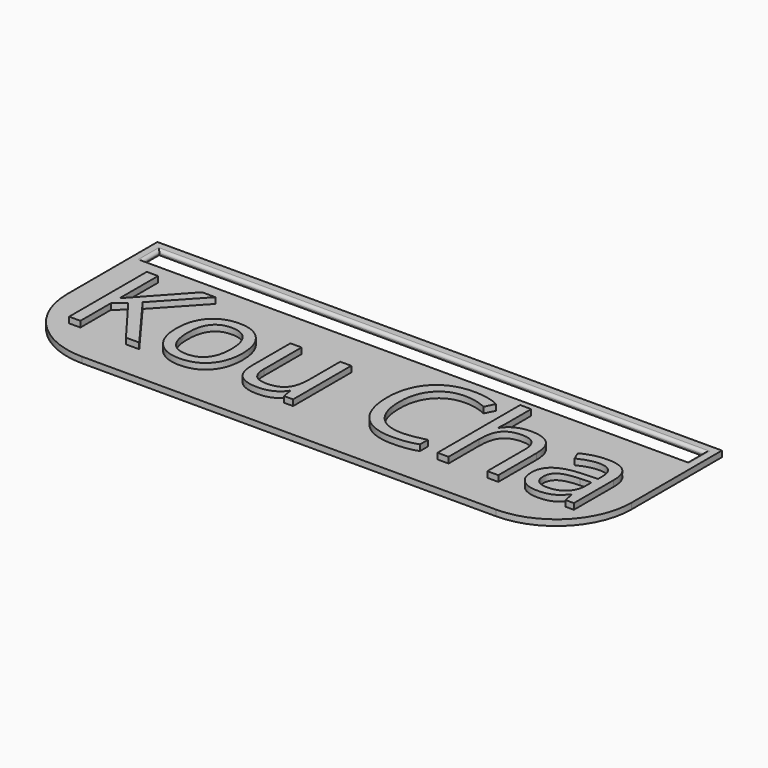
from build123d import *

# Parameters (mm, degrees)
F0_W         = 190.5
F0_H         = 63.5
F1_DEPTH     = 2
F2_W         = 183.896
F2_H         = 7.62
F3_DEPTH     = 25.4
F4_R         = 0.99999
F5_R         = 0.99999
F6_R         = 25.4
F7_TEXT_SIZE = 45.8709235296
F8_DEPTH     = 2


# Not quite as in the source:
# - a fillet or chamfer is up to 0.001 mm smaller than in the source, because OpenCascade refuses the exact size
# - Text() gives the source's letters only with a copy of the font that has no kerning and outlines rounded to 1/6400 em; it was checked with that copy


with BuildPart() as f1:
    # F0 (on Top) → F1 (new body)
    with BuildSketch(Plane.XY):
        with Locations((1.791532172, 31.75)):
            Rectangle(F0_W, F0_H)
    extrude(amount=F1_DEPTH)

    # F2 (on face) → F3 (cut)
    with BuildSketch(Plane.XY.offset(2)):
        with Locations((1.791532172, 56.388)):
            Rectangle(F2_W, F2_H)
    extrude(amount=-F3_DEPTH, mode=Mode.SUBTRACT)

    # F4 (radius 1 in the source; OpenCascade refuses exactly that, so slightly less here)
    f4_edges = [f1.edges().sort_by_distance(p)[0] for p in [
        (1.791532, 60.198, 2),
        (1.791532, 60.198, 0),
    ]]
    fillet(f4_edges, radius=F4_R)

    # F5 (radius 1 in the source; OpenCascade refuses exactly that, so slightly less here)
    f5_edges = [f1.edges().sort_by_distance(p)[0] for p in [
        (93.739532, 56.388, 0),
        (93.739532, 56.388, 2),
        (-90.156468, 56.388, 2),
        (-90.156468, 56.388, 0),
    ]]
    fillet(f5_edges, radius=F5_R)

    # F6
    f6_edges = [f1.edges().sort_by_distance(p)[0] for p in [
        (97.041532, 0, 1),
        (-93.458468, 0, 1),
    ]]
    fillet(f6_edges, radius=F6_R)

    # F7 (on face) → F8 (join)
    with BuildSketch(Plane.XY.offset(2)):
        with Locations((-87.108467828, 12.7)):
            Text('Kou Cha', F7_TEXT_SIZE, font='Open Sans', text_align=(TextAlign.LEFT, TextAlign.BOTTOM))
    extrude(amount=F8_DEPTH)


solid = f1.part
